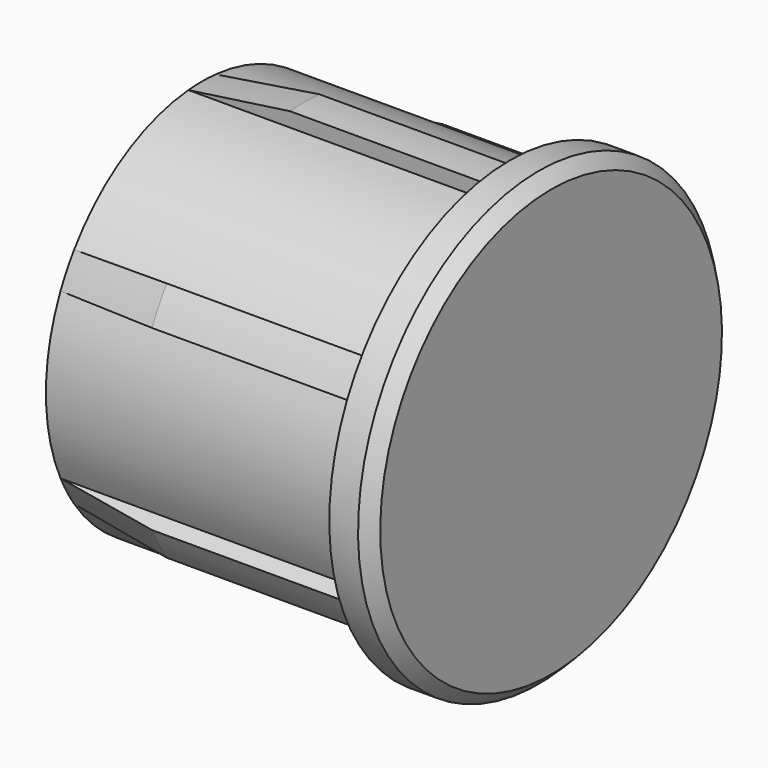
from build123d import *

# Parameters (mm, degrees)
F2_ANGLE_BACK   = 5
F2_ANGLE        = 10
F2_COPIES_COUNT = 6
F3_SIZE         = 0.6


# Not quite as in the source:
# - a pattern or mirror of a feature is missing from the dataset's text; its kind, count and spacing are read off the source's solid


with BuildPart() as f1:
    # F0 (on Front) → F1 (revolve)
    with BuildSketch(Plane.XZ):
        Polygon((-2, 0), (0, 0), (0, 11), (-2, 11), (-2, 10.25), (-2, 9.5), (-17, 9.5), (-17, 7), (-2, 7), align=None)
    revolve(axis=Axis((-8.5, 0, 0), (-1, 0, 0)))

    # F0 (on Front) → F2 (revolve)
    with BuildSketch(Plane.XZ, mode=Mode.PRIVATE) as f2_sk:
        Polygon((-2, 9.5), (-2, 10.25), (-12, 10.25), (-17, 9.5), align=None)
    f2 = revolve(f2_sk.sketch.rotate(Axis((-8.5, 0, 0), (-1, 0, 0)), -F2_ANGLE_BACK), axis=Axis((-8.5, 0, 0), (-1, 0, 0)), revolution_arc=F2_ANGLE)

    # F2_copies: F2 ×6 about axis
    f2_copies_axis = Axis((0, 0, 0), (1, 0, 0))
    for i in range(1, F2_COPIES_COUNT):
        add(f2.rotate(f2_copies_axis, i * 360 / F2_COPIES_COUNT))

    # F3
    f3_edges = [f1.edges().sort_by_distance(p)[0] for p in [
        (0, 0, -11),
    ]]
    chamfer(f3_edges, length=F3_SIZE)


solid = f1.part
